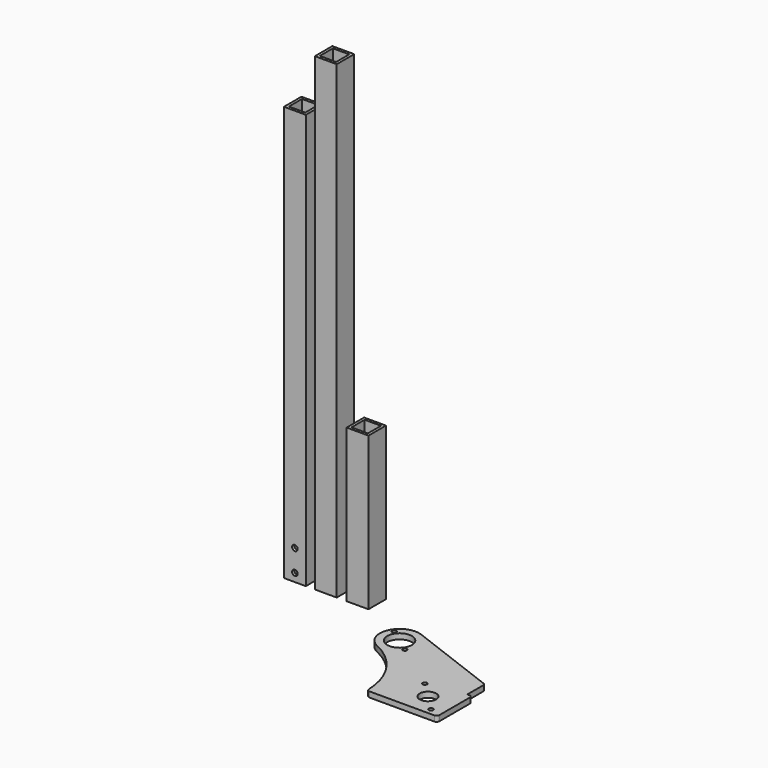
from build123d import *

# Parameters (mm, degrees)
F0_W     = 25.4
F0_H     = 25.4
F0_W_2   = 19.05
F0_H_2   = 19.05
F1_DEPTH = 482.6
F2_R     = 3.2385
F3_DEPTH = 25.4
F4_DEPTH = 546.1
F5_DEPTH = 177.8
F6_R     = 2.4765
F6_R_2   = 14.2875
F6_R_3   = 2.5527
F6_R_4   = 9.525
F7_DEPTH = 6.35
F8_R     = 3.175


# Not quite as in the source:
# - a length typed as a fraction of an inch, garbled in the dataset ("3 / 203.2 mm" for 3/8 in), is restored


with BuildPart() as f1:
    # F0 (on Top) → F1 (new body)
    with BuildSketch(Plane.XY):
        with Locations((-71.7274532759, 43.1469418108)):
            Rectangle(F0_W, F0_H)
        with Locations((-71.7274532759, 43.1469418108)):
            Rectangle(F0_W_2, F0_H_2, mode=Mode.SUBTRACT)
    extrude(amount=F1_DEPTH)

    # F2 (on face) → F3 (cut, through all)
    with BuildSketch(Plane.XZ.offset(-30.4469418108)):
        with Locations((-71.7274532759, 34.925)):
            Circle(F2_R)
        with Locations((-71.7274532759, 9.525)):
            Circle(F2_R)
    extrude(amount=-F3_DEPTH, mode=Mode.SUBTRACT)


with BuildPart() as f4:
    # F0 (on Top) → F4 (new body)
    with BuildSketch(Plane.XY):
        with Locations((-35.7863716781, 43.1469418108)):
            Rectangle(F0_W, F0_H)
        with Locations((-35.7863716781, 43.1469418108)):
            Rectangle(F0_W_2, F0_H_2, mode=Mode.SUBTRACT)
    extrude(amount=F4_DEPTH)


with BuildPart() as f5:
    # F0 (on Top) → F5 (new body)
    with BuildSketch(Plane.XY):
        with Locations((1.1303923199, 43.1469418108)):
            Rectangle(F0_W, F0_H)
        with Locations((1.1303923199, 43.1469418108)):
            Rectangle(F0_W_2, F0_H_2, mode=Mode.SUBTRACT)
    extrude(amount=F5_DEPTH)


with BuildPart() as f7:
    # F6 (on Top) → F7 (new body)
    with BuildSketch(Plane.XY):
        with BuildLine():
            Line((196.1707963228, -28.3818552375), (90.0035320812, 12.032559313))
            ThreePointArc((90.0035320812, 12.032559313), (60.7971369321, -0.4729343166), (72.2960630652, -30.0900845224))
            ThreePointArc((72.2960630652, -30.0900845224), (107.0316785467, -60.3610906142), (119.9707963228, -104.5818552375))
            Line((119.9707963228, -104.5818552375), (145.3707963228, -104.5818552375))
            Line((145.3707963228, -104.5818552375), (145.3707963228, -53.7818552375))
            Line((145.3707963228, -53.7818552375), (196.1707963228, -53.7818552375))
            Line((196.1707963228, -53.7818552375), (196.1707963228, -28.3818552375))
        make_face()
        with Locations((96.8203453355, -20.3007543763)):
            Circle(F6_R, mode=Mode.SUBTRACT)
        with Locations((81.8707963228, -9.3318552375)):
            Circle(F6_R_2, mode=Mode.SUBTRACT)
        with Locations((66.9212473101, 1.6370439013)):
            Circle(F6_R, mode=Mode.SUBTRACT)
        Polygon((201.7153054476, -53.7818552375), (196.1707963228, -53.7818552375), (145.3707963228, -53.7818552375), (145.3707963228, -104.5818552375), (201.7153054476, -104.5818552375), align=None)
        with Locations((188.6924888704, -97.1423674796)):
            Circle(F6_R_3, mode=Mode.SUBTRACT)
        with Locations((170.7319766283, -79.1818552375)):
            Circle(F6_R_4, mode=Mode.SUBTRACT)
        with Locations((152.7714643862, -61.2213429953)):
            Circle(F6_R_3, mode=Mode.SUBTRACT)
    extrude(amount=F7_DEPTH)

    # F8
    f8_edges = [f7.edges().sort_by_distance(p)[0] for p in [
        (196.170796, -28.381855, 3.175),
        (119.970796, -104.581855, 3.175),
        (201.715305, -53.781855, 3.175),
        (201.715305, -104.581855, 3.175),
    ]]
    fillet(f8_edges, radius=F8_R)


solid = Compound([f1.part, f4.part, f5.part, f7.part])
